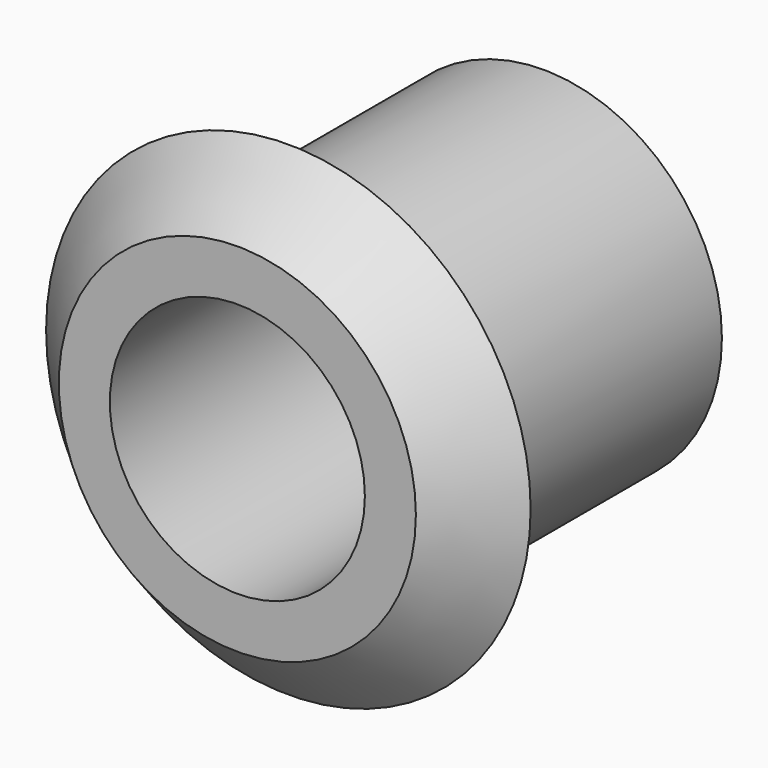
from build123d import *

# Parameters (mm, degrees)
F0_R     = 19
F0_R_2   = 14
F0_R_3   = 10
F1_DEPTH = 5
F2_DEPTH = 25
F3_SIZE  = 4.99999
F4_SIZE  = 2
F5_R     = 6.7


# Not quite as in the source:
# - a fillet or chamfer is up to 0.001 mm smaller than in the source, because OpenCascade refuses the exact size


with BuildPart() as f1:
    # F0 (on Front) → F1 (new body)
    with BuildSketch(Plane.XZ):
        Circle(F0_R)
        Circle(F0_R_2, mode=Mode.SUBTRACT)
        Circle(F0_R_2)
        Circle(F0_R_3, mode=Mode.SUBTRACT)
    extrude(amount=F1_DEPTH)

    # F0 (on Front) → F2 (join)
    with BuildSketch(Plane.XZ):
        Circle(F0_R_2)
        Circle(F0_R_3, mode=Mode.SUBTRACT)
    extrude(amount=-F2_DEPTH)

    # F3 (size 5 in the source; OpenCascade refuses exactly that, so slightly less here)
    f3_edges = [f1.edges().sort_by_distance(p)[0] for p in [
        (-19, -5, 0),
    ]]
    chamfer(f3_edges, length=F3_SIZE)

    # F4
    f4_edges = [f1.edges().sort_by_distance(p)[0] for p in [
        (-10, 25, 0),
    ]]
    chamfer(f4_edges, length=F4_SIZE)

    # F5
    f5_edges = [f1.edges().sort_by_distance(p)[0] for p in [
        (-10, 23, 0),
    ]]
    fillet(f5_edges, radius=F5_R)


solid = f1.part
